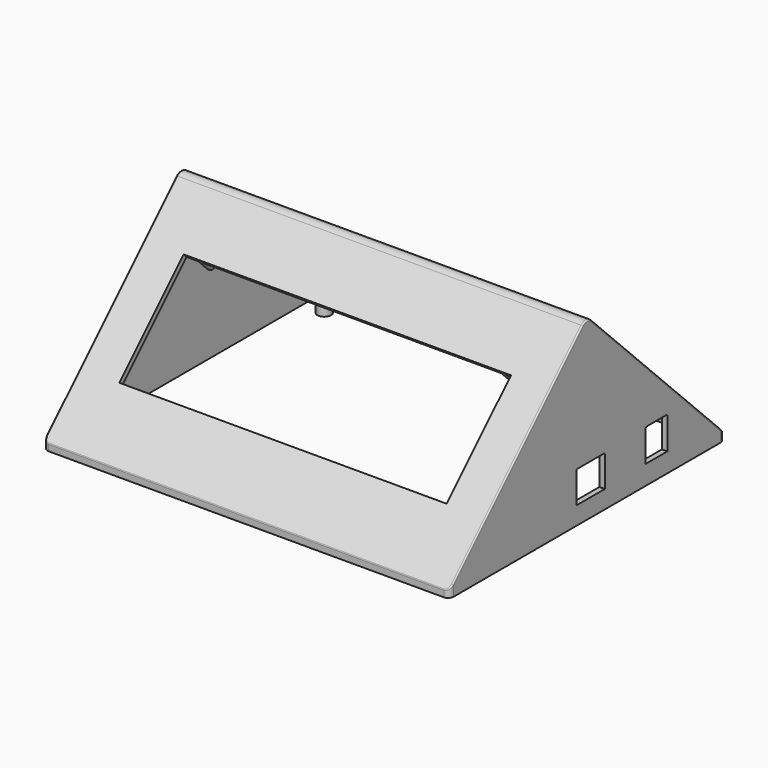
from build123d import *

# Parameters (mm, degrees)
F1_DEPTH  = 150
F2_T      = -2
F4_W      = 121
F4_H      = 42
F5_DEPTH  = 3
F6_R      = 3
F8_R      = 1.5
F8_R_2    = 0.75
F9_DEPTH  = 8.5
F10_R     = 2.5
F10_R_2   = 1.5
F12_R     = 2.5
F12_R_2   = 1.25
F13_REACH = 69.4690374315
F14_W     = 150
F14_H     = 127.2792206136
F14_W_2   = 146
F14_H_2   = 121.6223663641
F15_DEPTH = 2.5
F16_R     = 2.5
F16_R_2   = 1.25
F18_R     = 2
F19_R     = 0.5
F7_W      = 10
F7_H      = 12
F7_W_2    = 13.1
F7_H_2    = 11.7
F20_DEPTH = 3
F21_R     = 0.5
F22_R     = 0.5
F23_R     = 6.5
F24_DEPTH = 2.5
F25_R     = 2.5
F25_R_2   = 1.25
F26_DEPTH = 2.5
F27_R     = 2.5
F28_DEPTH = 1.5
F29_R     = 3


with BuildPart() as f1:
    # F0 (on Right) → F1 (new body)
    with BuildSketch(Plane.YZ):
        Polygon((63.6396103068, 63.6396103068), (0, 0), (127.2792206136, 0), align=None)
    extrude(amount=F1_DEPTH)

    # F2
    f2_openings = [f1.faces().sort_by_distance(p)[0] for p in [
        (75, 63.63961, 0),
    ]]
    offset(amount=F2_T, openings=f2_openings)

    # F4 (on offset) → F5 (cut)
    with BuildSketch(Plane(origin=(0, 0, 0), x_dir=(1, 0, 0), z_dir=(0, -0.7071067812, 0.7071067812))):
        with Locations((75, 45)):
            Rectangle(F4_W, F4_H)
    extrude(amount=-F5_DEPTH, mode=Mode.SUBTRACT)

    # F6
    f6_edges = [f1.edges().sort_by_distance(p)[0] for p in [
        (75, 63.63961, 63.63961),
    ]]
    fillet(f6_edges, radius=F6_R)

    # F8 (on face) → F9 (join)
    with BuildSketch(Plane(origin=(0, 0, 0), x_dir=(1, 0, 0), z_dir=(0, -0.7071067812, 0.7071067812))):
        with Locations((131, 67.5)):
            Circle(F8_R)
        with Locations((131, 67.5)):
            Circle(F8_R_2, mode=Mode.SUBTRACT)
        with Locations((131, 22.5)):
            Circle(F8_R)
        with Locations((131, 22.5)):
            Circle(F8_R_2, mode=Mode.SUBTRACT)
        with Locations((19, 67.5)):
            Circle(F8_R)
        with Locations((19, 67.5)):
            Circle(F8_R_2, mode=Mode.SUBTRACT)
        with Locations((19, 22.5)):
            Circle(F8_R)
        with Locations((19, 22.5)):
            Circle(F8_R_2, mode=Mode.SUBTRACT)
    extrude(amount=-F9_DEPTH)

    # F10 (on face) → F11 (join, up to the last surface of F1)
    with BuildSketch(Plane(origin=(0, 0, 0), x_dir=(1, 0, 0), z_dir=(0, 0, -1))):
        with Locations((10, -10)):
            Circle(F10_R)
        with Locations((10, -10)):
            Circle(F10_R_2, mode=Mode.SUBTRACT)
    extrude(until=Until.LAST, dir=(0, 0, 1))

    f13_end = Plane(origin=(75.2433178079, 33.3209918004, 30.4925646757), x_dir=(0, 0.7071067812, 0.7071067812), z_dir=(0, 0.7071067812, -0.7071067812))
    # F12 (on face) → F13 (join, up to a plane its end follows)
    with BuildSketch(Plane(origin=(0, 0, 0), x_dir=(1, 0, 0), z_dir=(0, 0, -1))):
        with Locations((10, -10)):
            Circle(F12_R)
        with Locations((10, -10)):
            Circle(F12_R_2, mode=Mode.SUBTRACT)
        with Locations((140, -10)):
            Circle(F12_R)
        with Locations((140, -10)):
            Circle(F12_R_2, mode=Mode.SUBTRACT)
    f13_long = extrude(amount=-F13_REACH, mode=Mode.PRIVATE)
    add(split(f13_long, bisect_by=f13_end, keep=Keep.TOP, mode=Mode.PRIVATE))

    # F14 (on face) → F15 (join)
    with BuildSketch(Plane(origin=(0, 0, 0), x_dir=(1, 0, 0), z_dir=(0, 0, -1))):
        with Locations((75, -63.6396103068)):
            Rectangle(F14_W, F14_H)
        with Locations((75, -63.6396103068)):
            Rectangle(F14_W_2, F14_H_2, mode=Mode.SUBTRACT)
    extrude(amount=F15_DEPTH)

    # F16 (on Top) → F17 (join, up to the next surface of F1)
    with BuildSketch(Plane.XY):
        with Locations((140, 117.279)):
            Circle(F16_R)
        with Locations((140, 117.279)):
            Circle(F16_R_2, mode=Mode.SUBTRACT)
        with Locations((10, 117.279)):
            Circle(F16_R)
        with Locations((10, 117.279)):
            Circle(F16_R_2, mode=Mode.SUBTRACT)
    extrude(until=Until.NEXT)

    # F18
    f18_edges = [f1.edges().sort_by_distance(p)[0] for p in [
        (150, 127.279221, -1.25),
        (150, 0, -1.25),
        (0, 0, -1.25),
        (0, 127.279221, -1.25),
    ]]
    fillet(f18_edges, radius=F18_R)

    # F19
    f19_edges = [f1.edges().sort_by_distance(p)[0] for p in [
        (0, 31.759145, 31.759145),
    ]]
    fillet(f19_edges, radius=F19_R)

    # F7 (on face) → F20 (cut)
    with BuildSketch(Plane.YZ.offset(150)):
        with Locations((95.7792206136, 10.65)):
            Rectangle(F7_W, F7_H)
        with Locations((65.3223664939, 10.0139604606)):
            Rectangle(F7_W_2, F7_H_2)
    extrude(amount=-F20_DEPTH, mode=Mode.SUBTRACT)

    # F21
    f21_edges = [f1.edges().sort_by_distance(p)[0] for p in [
        (149, 90.779221, 16.65),
        (149, 100.779221, 16.65),
    ]]
    fillet(f21_edges, radius=F21_R)

    # F22
    f22_edges = [f1.edges().sort_by_distance(p)[0] for p in [
        (149, 71.872366, 15.86396),
        (149, 58.772366, 15.86396),
    ]]
    fillet(f22_edges, radius=F22_R)

    # F23 (on face) → F24 (cut)
    with BuildSketch(Plane(origin=(0, 0, 0), x_dir=(0, -1, 0), z_dir=(-1, 0, 0))):
        with Locations((-64, 47.5)):
            Circle(F23_R)
    extrude(amount=-F24_DEPTH, mode=Mode.SUBTRACT)

    # F25 (on face) → F26 (join)
    with BuildSketch(Plane(origin=(0, 0, 0), x_dir=(1, 0, 0), z_dir=(0, 0, -1))):
        with Locations((10, -10)):
            Circle(F25_R)
        with Locations((10, -10)):
            Circle(F25_R_2, mode=Mode.SUBTRACT)
        with Locations((140, -10)):
            Circle(F25_R)
        with Locations((140, -10)):
            Circle(F25_R_2, mode=Mode.SUBTRACT)
        with Locations((10, -117.279)):
            Circle(F25_R)
        with Locations((10, -117.279)):
            Circle(F25_R_2, mode=Mode.SUBTRACT)
        with Locations((140, -117.279)):
            Circle(F25_R)
        with Locations((140, -117.279)):
            Circle(F25_R_2, mode=Mode.SUBTRACT)
    extrude(amount=F26_DEPTH)

    # F27 (on face) → F28 (cut)
    with BuildSketch(Plane(origin=(0, 0, 0), x_dir=(0, -1, 0), z_dir=(-1, 0, 0))):
        with Locations((-64, 32.5)):
            Circle(F27_R)
    extrude(amount=-F28_DEPTH, mode=Mode.SUBTRACT)

    # F29
    f29_edges = [f1.edges().sort_by_distance(p)[0] for p in [
        (75, 63.63961, 60.811183),
    ]]
    fillet(f29_edges, radius=F29_R)


solid = f1.part
